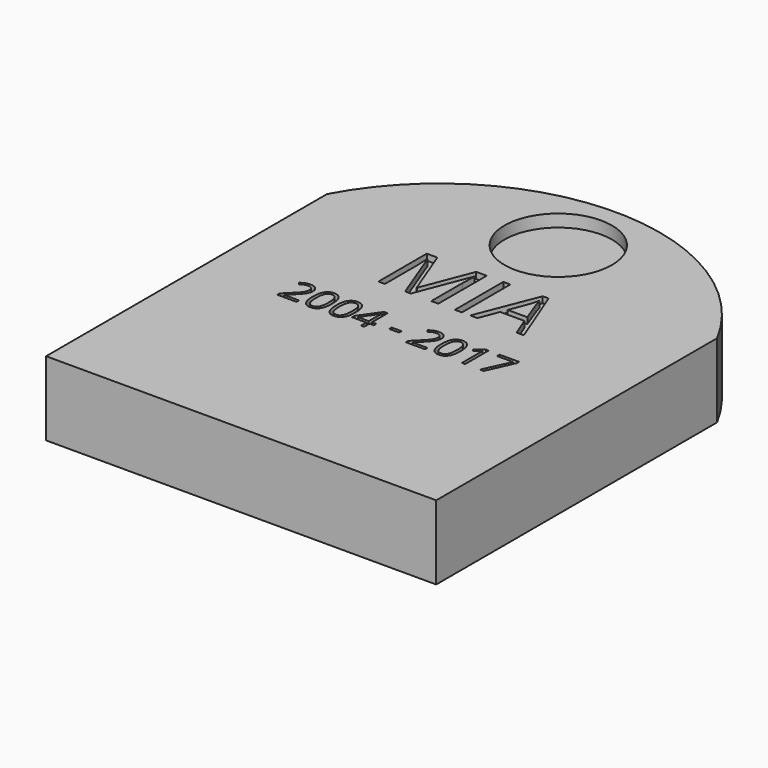
from build123d import *

# Parameters (mm, degrees)
F0_W         = 200
F0_H         = 180
F1_DEPTH     = 38
F2_TEXT_SIZE = 43.4440457159
F3_DEPTH     = 3.175
F4_R         = 27.5149084124
F5_DEPTH     = 6.35
F6_TEXT_SIZE = 21.0527527556
F7_DEPTH     = 3.175


# Not quite as in the source:
# - Text() gives the source's letters only with a copy of the font that has no kerning and outlines rounded to 1/6400 em; it was checked with that copy


with BuildPart() as f1:
    # F0 (on Top) → F1 (new body)
    with BuildSketch(Plane.XY):
        with BuildLine():
            ThreePointArc((116.6089320848, 109.0135069191), (16.6089320848, 169.0135069191), (-83.3910679152, 109.0135069191))
            Line((-83.3910679152, 109.0135069191), (116.6089320848, 109.0135069191))
        make_face()
        with Locations((16.6089320848, 19.0135069191)):
            Rectangle(F0_W, F0_H)
    extrude(amount=F1_DEPTH)

    # F2 (on face) → F3 (cut)
    with BuildSketch(Plane.XY.offset(38)):
        with Locations((-24.2115005577, 62.6507401466)):
            Text('MIA', F2_TEXT_SIZE, font='Open Sans', text_align=(TextAlign.LEFT, TextAlign.BOTTOM))
    extrude(amount=-F3_DEPTH, mode=Mode.SUBTRACT)

    # F4 (on face) → F5 (cut)
    with BuildSketch(Plane.XY.offset(38)):
        with Locations((16.6089320848, 132.2135069191)):
            Circle(F4_R)
    extrude(amount=-F5_DEPTH, mode=Mode.SUBTRACT)

    # F6 (on face) → F7 (cut)
    with BuildSketch(Plane.XY.offset(38)):
        with Locations((-45.4008827651, 28.4427581626)):
            Text('2004 - 2017', F6_TEXT_SIZE, font='Open Sans', text_align=(TextAlign.LEFT, TextAlign.BOTTOM))
    extrude(amount=-F7_DEPTH, mode=Mode.SUBTRACT)


solid = f1.part
